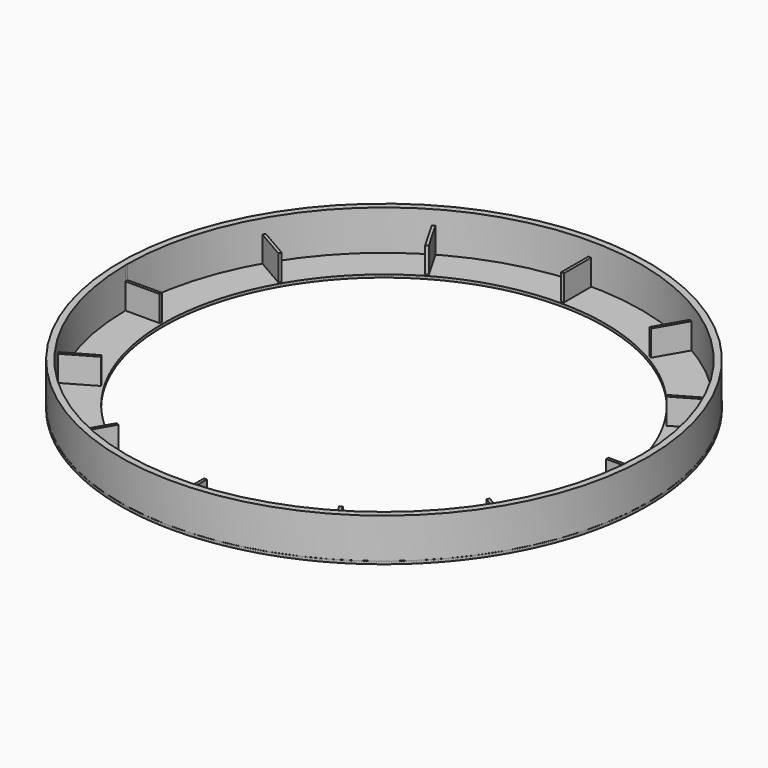
from build123d import *

# Parameters (mm, degrees)
F0_R     = 92.5
F0_R_2   = 77.5
F1_DEPTH = 1
F3_DEPTH = 9
F5_COUNT = 12
F2_R     = 92.5
F6_DEPTH = 14


# Not quite as in the source:
# - the program builds the solid bodies; features that only make, move or delete a surface that nothing else refers to are left out


with BuildPart() as f1:
    # F0 (on Top) → F1 (new body)
    with BuildSketch(Plane.XY):
        Circle(F0_R)
        Circle(F0_R_2, mode=Mode.SUBTRACT)
    extrude(amount=F1_DEPTH)

    # F2 (on face) → F3 (join)
    with BuildSketch(Plane.XY.offset(1)):
        with BuildLine():
            Line((-78.2484025396, 0.5), (-90.2486149478, 0.5))
            ThreePointArc((-90.2486149478, 0.5), (-90.25, 0), (-90.2486149478, -0.5))
            Line((-90.2486149478, -0.5), (-78.2484025396, -0.5))
            ThreePointArc((-78.2484025396, -0.5), (-78.25, 0), (-78.2484025396, 0.5))
        make_face()
    extrude(amount=F3_DEPTH)


with BuildPart() as f5_1:
    # F5: instance of F1
    add(f1.part.rotate(Axis((0, 0, -0.5706530064), (0, 0, 1)), 1 * 360 / F5_COUNT))


with BuildPart() as f5_2:
    # F5: instance of F1
    add(f1.part.rotate(Axis((0, 0, -0.5706530064), (0, 0, 1)), 2 * 360 / F5_COUNT))


with BuildPart() as f5_3:
    # F5: instance of F1
    add(f1.part.rotate(Axis((0, 0, -0.5706530064), (0, 0, 1)), 3 * 360 / F5_COUNT))


with BuildPart() as f5_4:
    # F5: instance of F1
    add(f1.part.rotate(Axis((0, 0, -0.5706530064), (0, 0, 1)), 4 * 360 / F5_COUNT))


with BuildPart() as f5_5:
    # F5: instance of F1
    add(f1.part.rotate(Axis((0, 0, -0.5706530064), (0, 0, 1)), 5 * 360 / F5_COUNT))


with BuildPart() as f5_6:
    # F5: instance of F1
    add(f1.part.rotate(Axis((0, 0, -0.5706530064), (0, 0, 1)), 6 * 360 / F5_COUNT))


with BuildPart() as f5_7:
    # F5: instance of F1
    add(f1.part.rotate(Axis((0, 0, -0.5706530064), (0, 0, 1)), 7 * 360 / F5_COUNT))


with BuildPart() as f5_8:
    # F5: instance of F1
    add(f1.part.rotate(Axis((0, 0, -0.5706530064), (0, 0, 1)), 8 * 360 / F5_COUNT))


with BuildPart() as f5_9:
    # F5: instance of F1
    add(f1.part.rotate(Axis((0, 0, -0.5706530064), (0, 0, 1)), 9 * 360 / F5_COUNT))


with BuildPart() as f5_10:
    # F5: instance of F1
    add(f1.part.rotate(Axis((0, 0, -0.5706530064), (0, 0, 1)), 10 * 360 / F5_COUNT))


with BuildPart() as f5_11:
    # F5: instance of F1
    add(f1.part.rotate(Axis((0, 0, -0.5706530064), (0, 0, 1)), 11 * 360 / F5_COUNT))


with BuildPart() as f6:
    # F2 (on face) → F6 (new body)
    with BuildSketch(Plane.XY.offset(1)):
        Circle(F2_R)
        with BuildLine():
            ThreePointArc((-90.2486149478, 0.5), (0.2500009592, 90.2496537363), (90.25, 0))
            ThreePointArc((90.25, 0), (0.2500009592, -90.2496537363), (-90.2486149478, -0.5))
            ThreePointArc((-90.2486149478, -0.5), (-90.25, 0), (-90.2486149478, 0.5))
        make_face(mode=Mode.SUBTRACT)
    extrude(amount=F6_DEPTH)


solid = Compound([f1.part, f5_1.part, f5_2.part, f5_3.part, f5_4.part, f5_5.part, f5_6.part, f5_7.part, f5_8.part, f5_9.part, f5_10.part, f5_11.part, f6.part])
